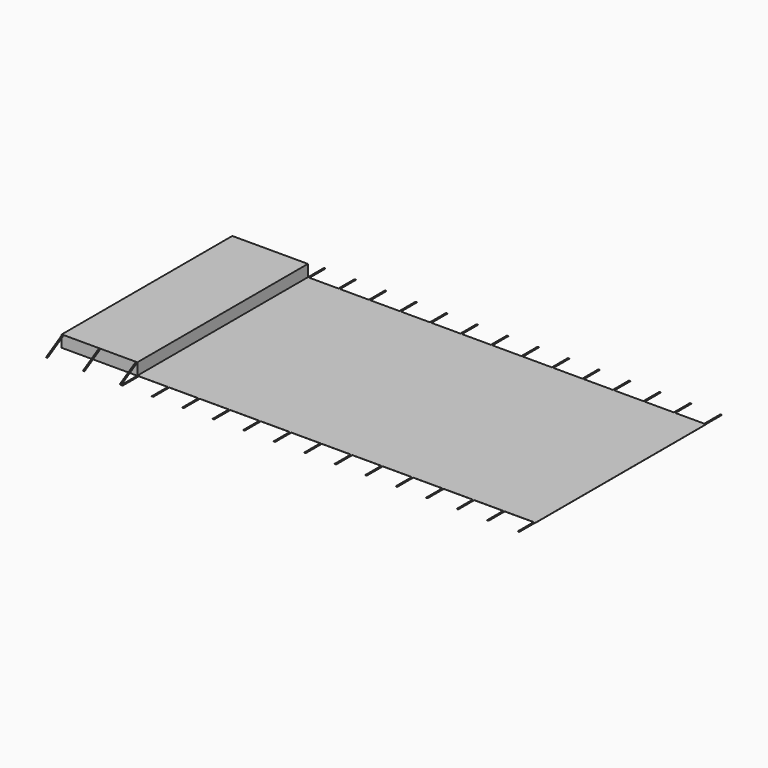
from build123d import *

# Parameters (mm, degrees)
F0_W     = 1500
F0_H     = 4230
F1_DEPTH = 235
F2_W     = 7900
F2_H     = 4230
F3_DEPTH = 2
F4_W     = 30
F4_H     = 400
F5_DEPTH = 2
F7_W     = 30
F7_H     = 463.9202661871
F8_DEPTH = 2


with BuildPart() as f1:
    # F0 (on Top) → F1 (new body)
    with BuildSketch(Plane.XY):
        with Locations((-799.7552353144, 1834.9275854864)):
            Rectangle(F0_W, F0_H)
    extrude(amount=F1_DEPTH)

    # F2 (on Top) → F3 (join)
    with BuildSketch(Plane.XY):
        with Locations((3900.2447646856, 1834.9275854864)):
            Rectangle(F2_W, F2_H)
    extrude(amount=F3_DEPTH)

    # F4 (on Top) → F5 (join)
    with BuildSketch(Plane.XY):
        with Locations((-34.7552353144, 4149.9275854864)):
            Rectangle(F4_W, F4_H)
        with Locations((570.2447646856, 4149.9275854864)):
            Rectangle(F4_W, F4_H)
        with Locations((1175.2447646856, 4149.9275854864)):
            Rectangle(F4_W, F4_H)
        with Locations((1780.2447646856, 4149.9275854864)):
            Rectangle(F4_W, F4_H)
        with Locations((2385.2447646856, 4149.9275854864)):
            Rectangle(F4_W, F4_H)
        with Locations((2990.2447646856, 4149.9275854864)):
            Rectangle(F4_W, F4_H)
        with Locations((3595.2447646856, 4149.9275854864)):
            Rectangle(F4_W, F4_H)
        with Locations((4200.2447646856, 4149.9275854864)):
            Rectangle(F4_W, F4_H)
        with Locations((4805.2447646856, 4149.9275854864)):
            Rectangle(F4_W, F4_H)
        with Locations((5410.2447646856, 4149.9275854864)):
            Rectangle(F4_W, F4_H)
        with Locations((6015.2447646856, 4149.9275854864)):
            Rectangle(F4_W, F4_H)
        with Locations((6620.2447646856, 4149.9275854864)):
            Rectangle(F4_W, F4_H)
        with Locations((7225.2447646856, 4149.9275854864)):
            Rectangle(F4_W, F4_H)
        with Locations((7830.2447646856, 4149.9275854864)):
            Rectangle(F4_W, F4_H)
        with Locations((-34.7552353144, -480.0724145136)):
            Rectangle(F4_W, F4_H)
        with Locations((570.2447646856, -480.0724145136)):
            Rectangle(F4_W, F4_H)
        with Locations((1780.2447646856, -480.0724145136)):
            Rectangle(F4_W, F4_H)
        with Locations((7225.2447646856, -480.0724145136)):
            Rectangle(F4_W, F4_H)
        with Locations((4805.2447646856, -480.0724145136)):
            Rectangle(F4_W, F4_H)
        with Locations((3595.2447646856, -480.0724145136)):
            Rectangle(F4_W, F4_H)
        with Locations((2385.2447646856, -480.0724145136)):
            Rectangle(F4_W, F4_H)
        with Locations((5410.2447646856, -480.0724145136)):
            Rectangle(F4_W, F4_H)
        with Locations((7830.2447646856, -480.0724145136)):
            Rectangle(F4_W, F4_H)
        with Locations((6620.2447646856, -480.0724145136)):
            Rectangle(F4_W, F4_H)
        with Locations((6015.2447646856, -480.0724145136)):
            Rectangle(F4_W, F4_H)
        with Locations((2990.2447646856, -480.0724145136)):
            Rectangle(F4_W, F4_H)
        with Locations((4200.2447646856, -480.0724145136)):
            Rectangle(F4_W, F4_H)
        with Locations((1175.2447646856, -480.0724145136)):
            Rectangle(F4_W, F4_H)
    extrude(amount=F5_DEPTH)

    # F7 (on 3pt) → F8 (join)
    with BuildSketch(Plane(origin=(0, -173.1626509598, 297.2749372701), x_dir=(1, 0, 0), z_dir=(0, 0.5033336687, -0.8640921351))):
        with Locations((-64.7552353144, 355.6850915907)):
            Rectangle(F7_W, F7_H)
        with Locations((-794.7552353144, 355.6850915907)):
            Rectangle(F7_W, F7_H)
        with Locations((-1524.7552353144, 355.6850915907)):
            Rectangle(F7_W, F7_H)
    extrude(amount=F8_DEPTH)


solid = f1.part
